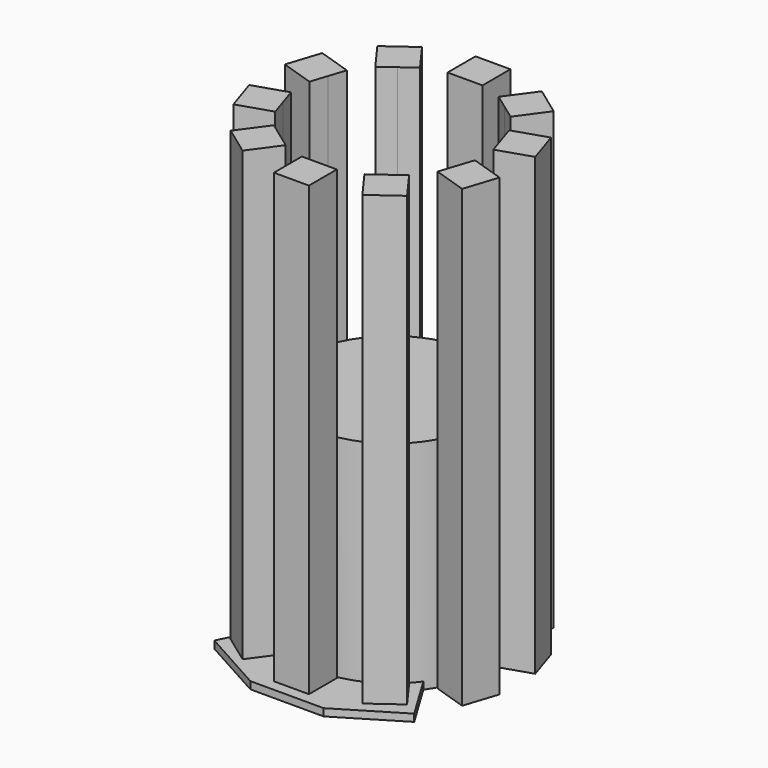
from build123d import *

# Parameters (mm, degrees)
F1_DEPTH = 120
F2_DEPTH = 250
F4_DEPTH = 4


# Not quite as in the source:
# - a feature names something its author has since deleted; it is built from what else it names


with BuildPart() as f1:
    # F0 (on Top) → F1 (new body)
    with BuildSketch(Plane.XY):
        with BuildLine():
            ThreePointArc((47.5528258507, -15.4508496082), (49.3844170388, -7.8217231946), (50, 0))
            ThreePointArc((50, 0), (49.3844170388, 7.8217231946), (47.5528258507, 15.4508496082))
            ThreePointArc((47.5528258507, 15.4508496082), (40.4508495047, 29.3892629092), (29.3892619315, 40.450850215))
            ThreePointArc((29.3892619315, 40.450850215), (15.4508493172, 47.5528259452), (0, 50))
            ThreePointArc((0, 50), (-15.450849525, 47.5528258777), (-29.389262285, 40.4508499582))
            ThreePointArc((-29.389262285, 40.4508499582), (-40.4508495406, 29.3892628598), (-47.5528257534, 15.4508499077))
            ThreePointArc((-47.5528257534, 15.4508499077), (-50, 5.095e-07), (-47.5528260682, -15.4508489386))
            ThreePointArc((-47.5528260682, -15.4508489386), (-40.4508501628, -29.3892620034), (-29.3892631734, -40.4508493128))
            ThreePointArc((-29.3892631734, -40.4508493128), (-15.4508500472, -47.552825708), (0, -50))
            ThreePointArc((0, -50), (15.4508493172, -47.5528259452), (29.3892619315, -40.4508502151))
            ThreePointArc((29.3892619315, -40.4508502151), (40.4508495047, -29.3892629092), (47.5528258507, -15.4508496082))
        make_face()
    extrude(amount=F1_DEPTH)

    # F0 (on Top) → F2 (join)
    with BuildSketch(Plane.XY):
        Polygon((-21.6226994686, -46.0935881408), (-29.3892631734, -40.4508493128), (-37.1558257606, -34.8081112967), (-48.4413026046, -50.3412375887), (-32.9081763126, -61.6267144328), align=None)
        Polygon((-44.5862626688, -24.5809922752), (-47.5528260682, -15.4508489386), (-50.5193889608, -6.3207071623), (-68.7796740736, -12.2538334543), (-62.8465477816, -30.5141185672), align=None)
        Polygon((9.6, -50), (0, -50), (-9.6, -50), (-9.6, -69.2), (9.6, -69.2), align=None)
        Polygon((37.1558257606, -34.8081112967), (29.3892619315, -40.4508502151), (21.6226994686, -46.0935881408), (32.9081763126, -61.6267144328), (48.4413026046, -50.3412375887), align=None)
        Polygon((50.5193889608, -6.3207071623), (47.5528258507, -15.4508496082), (44.5862626688, -24.5809922752), (62.8465477816, -30.5141185672), (68.7796740736, -12.2538334543), align=None)
        Polygon((44.5862626688, 24.5809922752), (47.5528258507, 15.4508496082), (50.5193889608, 6.3207071623), (68.7796740736, 12.2538334543), (62.8465477816, 30.5141185672), align=None)
        Polygon((21.6226994686, 46.0935881408), (29.3892619315, 40.450850215), (37.1558257606, 34.8081112967), (48.4413026046, 50.3412375887), (32.9081763126, 61.6267144328), align=None)
        Polygon((-9.6, 50), (0, 50), (9.6, 50), (9.6, 69.2), (-9.6, 69.2), align=None)
        Polygon((-37.1558257606, 34.8081112967), (-29.389262285, 40.4508499582), (-21.6226994686, 46.0935881408), (-32.9081763126, 61.6267144328), (-48.4413026046, 50.3412375887), align=None)
        Polygon((-50.5193889608, 6.3207071623), (-47.5528257534, 15.4508499077), (-44.5862626688, 24.5809922752), (-62.8465477816, 30.5141185672), (-68.7796740736, 12.2538334543), align=None)
    extrude(amount=F2_DEPTH)


with BuildPart() as f4:
    # F3 (on Top) → F4 (new body)
    with BuildSketch(Plane.XY):
        with BuildLine():
            ThreePointArc((-36.5395719078, -34.1300407969), (-38.5003757753, -31.9017407858), (-40.3255031982, -29.5610181119))
            Line((-40.3255031982, -29.5610181119), (-40.8250220898, -30.5666087646))
            Line((-40.8250220898, -30.5666087646), (-53.2520930962, -55.5837735933))
            Line((-53.2520930962, -55.5837735933), (-17.6129629184, -75.3755012347))
            Line((-17.6129629184, -75.3755012347), (22.63964626, -75.3755012347))
            Line((22.63964626, -75.3755012347), (56.161962921, -55.0787862979))
            Line((56.161962921, -55.0787862979), (41.0978779096, -30.1987488371))
            Line((41.0978779096, -30.1987488371), (40.5363164273, -29.2712666365))
            ThreePointArc((40.5363164273, -29.2712666365), (38.646780385, -31.7242236449), (36.6090363432, -34.0555202283))
            Line((36.6090363432, -34.0555202283), (37.1558257606, -34.8081112967))
            Line((37.1558257606, -34.8081112967), (37.2077401251, -34.8795652895))
            Line((37.2077401251, -34.8795652895), (48.4413026046, -50.3412375887))
            Line((48.4413026046, -50.3412375887), (32.9081763126, -61.6267144328))
            Line((32.9081763126, -61.6267144328), (21.6746138331, -46.1650421335))
            Line((21.6746138331, -46.1650421335), (21.6226994686, -46.0935881408))
            Line((21.6226994686, -46.0935881408), (21.0759100512, -45.3409970723))
            ThreePointArc((21.0759100512, -45.3409970723), (15.4508497187, -47.5528258148), (9.6, -49.0697462802))
            Line((9.6, -49.0697462802), (9.6, -50))
            Line((9.6, -50), (9.6, -69.2))
            Line((9.6, -69.2), (-9.6, -69.2))
            Line((-9.6, -69.2), (-9.6, -50))
            Line((-9.6, -50), (-9.6, -49.0697462802))
            ThreePointArc((-9.6, -49.0697462802), (-15.4508497187, -47.5528258148), (-21.0759100512, -45.3409970723))
            Line((-21.0759100512, -45.3409970723), (-21.6226994686, -46.0935881408))
            Line((-21.6226994686, -46.0935881408), (-21.6746138331, -46.1650421335))
            Line((-21.6746138331, -46.1650421335), (-32.9081763126, -61.6267144328))
            Line((-32.9081763126, -61.6267144328), (-48.4413026046, -50.3412375887))
            Line((-48.4413026046, -50.3412375887), (-37.2077401251, -34.8795652895))
            Line((-37.2077401251, -34.8795652895), (-37.1558257606, -34.8081112967))
            Line((-37.1558257606, -34.8081112967), (-36.5395719078, -34.1300407969))
        make_face()
    extrude(amount=F4_DEPTH)


solid = Compound([f1.part, f4.part])
